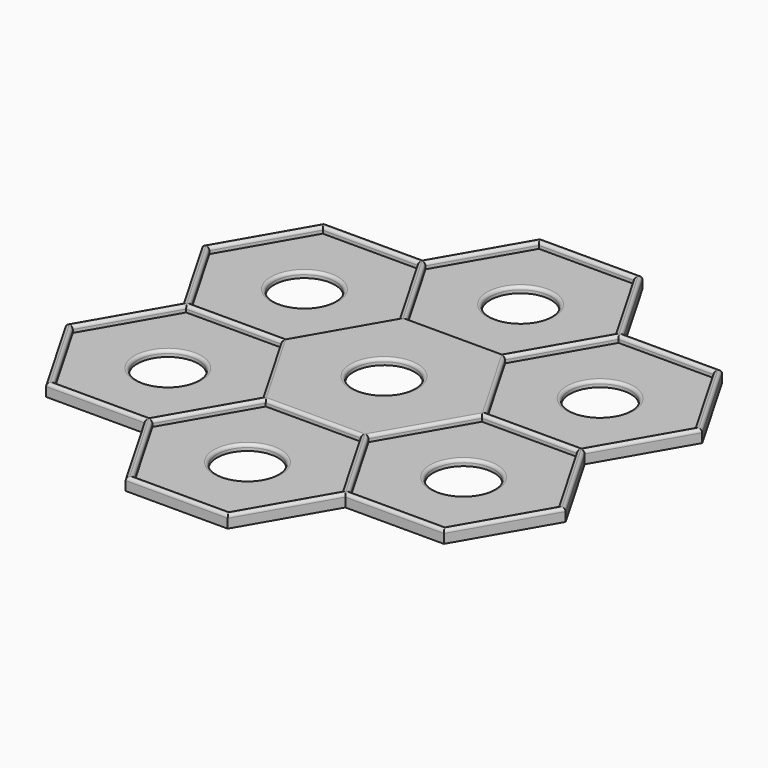
from build123d import *

# Parameters (mm, degrees)
F0_R     = 10
F1_DEPTH = 2
F2_DEPTH = 4
F3_R     = 0.99999
F4_START = 2
F4_DEPTH = 2
F5_R     = 1


# Not quite as in the source:
# - two fillets or chamfers of one size are made in one step
# - a fillet or chamfer is up to 0.001 mm smaller than in the source, because OpenCascade refuses the exact size


with BuildPart() as f1:
    # F0 (on Top) → F1 (new body)
    with BuildSketch(Plane.XY):
        Polygon((-64.0859146607, 54.9999594737), (-79.6743548546, 27.999949616), (-64.0858805124, 0.9999594737), (-32.9089659762, 0.9999791892), (-17.3205257822, 27.9999890469), (-32.9090001244, 54.9999791892), align=None)
        with Locations((-48.4974403184, 27.9999693314)):
            Circle(F0_R, mode=Mode.SUBTRACT)
    extrude(amount=F1_DEPTH)



with BuildPart() as f1b:
    # F0 (on Top) → F1, piece 2 (new body)
    with BuildSketch(Plane.XY):
        Polygon((-15.5885097552, 82.9999901422), (-31.1769499492, 55.9999802845), (-15.588475607, 28.9999901422), (15.5884389292, 29.0000098577), (31.1768791232, 56.0000197155), (15.588404781, 83.0000098577), align=None)
        with Locations((-3.5413e-05, 56)):
            Circle(F0_R, mode=Mode.SUBTRACT)
    extrude(amount=F1_DEPTH)


with BuildPart() as f1c:
    # F0 (on Top) → F1, piece 3 (new body)
    with BuildSketch(Plane.XY):
        Polygon((32.9089305632, 55.0000208108), (17.3204903692, 28.000010953), (32.9089647114, 1.0000208108), (64.0858792477, 1.0000405263), (79.6743194417, 28.000050384), (64.0858450994, 55.0000405263), align=None)
        with Locations((48.4974049054, 28.0000306685)):
            Circle(F0_R, mode=Mode.SUBTRACT)
    extrude(amount=F1_DEPTH)


with BuildPart() as f1d:
    # F0 (on Top) → F1, piece 4 (new body)
    with BuildSketch(Plane.XY):
        Polygon((32.9089659762, -0.9999791892), (17.3205257822, -27.9999890469), (32.9090001244, -54.9999791892), (64.0859146607, -54.9999594737), (79.6743548546, -27.999949616), (64.0858805124, -0.9999594737), align=None)
        with Locations((48.4974403184, -27.9999693314)):
            Circle(F0_R, mode=Mode.SUBTRACT)
    extrude(amount=F1_DEPTH)


with BuildPart() as f1e:
    # F0 (on Top) → F1, piece 5 (new body)
    with BuildSketch(Plane.XY):
        Polygon((-15.5884389292, -29.0000098577), (-31.1768791232, -56.0000197155), (-15.588404781, -83.0000098577), (15.5885097552, -82.9999901422), (31.1769499492, -55.9999802845), (15.588475607, -28.9999901422), align=None)
        with Locations((3.5413e-05, -56)):
            Circle(F0_R, mode=Mode.SUBTRACT)
    extrude(amount=F1_DEPTH)


with BuildPart() as f1f:
    # F0 (on Top) → F1, piece 6 (new body)
    with BuildSketch(Plane.XY):
        Polygon((-64.0858792477, -1.0000405263), (-79.6743194417, -28.000050384), (-64.0858450994, -55.0000405263), (-32.9089305632, -55.0000208108), (-17.3204903692, -28.000010953), (-32.9089647114, -1.0000208108), align=None)
        with Locations((-48.4974049054, -28.0000306685)):
            Circle(F0_R, mode=Mode.SUBTRACT)
    extrude(amount=F1_DEPTH)


with BuildPart() as f1_1:
    add(f1.part)

    add(f1b.part)  # F2 merges F1b

    add(f1c.part)  # F2 merges F1c

    add(f1d.part)  # F2 merges F1d

    add(f1e.part)  # F2 merges F1e

    add(f1f.part)  # F2 merges F1f
    # F0 (on Top) → F2 (join)
    with BuildSketch(Plane.XY):
        Polygon((-81.9837559314, 27.9999481555), (-65.8179547179, 0), (-81.9837445487, -28.0000102228), (-65.2405443731, -57.0000412565), (-32.9089292984, -57.0000208108), (-16.7431040546, -85.0000105879), (16.7432115584, -84.999989412), (32.9090013892, -56.9999791892), (65.2406164638, -56.9999587435), (81.9837559314, -27.9999481555), (65.8179306876, 4.16216e-05), (81.9837205184, 28.0000518444), (65.2405443731, 57.0000412565), (32.9089292984, 57.0000208108), (16.7431040546, 85.0000105879), (-16.7432115584, 84.999989412), (-32.9090013892, 56.9999791892), (-65.2406164638, 56.9999587435), align=None)
        Polygon((-64.0858450994, -55.0000405263), (-79.6743194417, -28.000050384), (-64.0858792477, -1.0000405263), (-32.9089647114, -1.0000208108), (-17.3204903692, -28.000010953), (-32.9089305632, -55.0000208108), align=None, mode=Mode.SUBTRACT)
        Polygon((-15.5884743422, 26.9999901422), (15.588440194, 27.0000098577), (31.1769145362, 1.97155e-05), (15.5884743422, -26.9999901422), (-15.588440194, -27.0000098577), (-31.1769145362, -1.97155e-05), align=None, mode=Mode.SUBTRACT)
        Polygon((-15.588404781, -83.0000098577), (-31.1768791232, -56.0000197155), (-15.5884389292, -29.0000098577), (15.588475607, -28.9999901422), (31.1769499492, -55.9999802845), (15.5885097552, -82.9999901422), align=None, mode=Mode.SUBTRACT)
        Polygon((32.9090001244, -54.9999791892), (17.3205257822, -27.9999890469), (32.9089659762, -0.9999791892), (64.0858805124, -0.9999594737), (79.6743548546, -27.999949616), (64.0859146607, -54.9999594737), align=None, mode=Mode.SUBTRACT)
        Polygon((-64.0858805124, 0.9999594737), (-79.6743548546, 27.999949616), (-64.0859146607, 54.9999594737), (-32.9090001244, 54.9999791892), (-17.3205257822, 27.9999890469), (-32.9089659762, 0.9999791892), align=None, mode=Mode.SUBTRACT)
        Polygon((-15.588475607, 28.9999901422), (-31.1769499492, 55.9999802845), (-15.5885097552, 82.9999901422), (15.588404781, 83.0000098577), (31.1768791232, 56.0000197155), (15.5884389292, 29.0000098577), align=None, mode=Mode.SUBTRACT)
        Polygon((32.9089647114, 1.0000208108), (17.3204903692, 28.000010953), (32.9089305632, 55.0000208108), (64.0858450994, 55.0000405263), (79.6743194417, 28.000050384), (64.0858792477, 1.0000405263), align=None, mode=Mode.SUBTRACT)
    extrude(amount=F2_DEPTH)

    # F3 (radius 1 in the source; OpenCascade refuses exactly that, so slightly less here)
    f3_edges = [f1_1.edges().sort_by_distance(p)[0] for p in [
        (-9.999965, -56, 2),
        (-58.497405, -28.000031, 2),
        (-58.49744, 27.999969, 2),
        (-10.000035, 56, 2),
        (38.497405, 28.000031, 2),
        (38.49744, -27.999969, 2),
        (-48.497422, -1.000031, 4),
        (-71.880099, -14.500045, 4),
        (-71.880082, -41.500045, 4),
        (-48.497388, -55.000031, 4),
        (-25.11471, -41.500016, 4),
        (-25.114728, -14.500016, 4),
        (24.826017, 71.000016, 4),
        (-5.4e-05, 85, 4),
        (-24.826106, 70.999984, 4),
        (-49.074809, 56.999969, 4),
        (-73.612186, 42.499953, 4),
        (-73.900855, 13.999974, 4),
        (-73.90085, -14.000005, 4),
        (-73.612144, -42.500026, 4),
        (-49.074737, -57.000031, 4),
        (-24.826017, -71.000016, 4),
        (5.4e-05, -85, 4),
        (24.826106, -70.999984, 4),
        (49.074809, -56.999969, 4),
        (73.612186, -42.499953, 4),
        (73.900843, -13.999953, 4),
        (73.900826, 14.000047, 4),
        (73.612132, 42.500047, 4),
        (49.074737, 57.000031, 4),
        (-23.382642, -69.500015, 4),
        (-23.382659, -42.500015, 4),
        (1.8e-05, -29, 4),
        (23.382713, -42.499985, 4),
        (23.38273, -69.499985, 4),
        (5.2e-05, -83, 4),
        (71.880135, -41.499955, 4),
        (48.497457, -54.999969, 4),
        (25.114763, -41.499984, 4),
        (25.114746, -14.499984, 4),
        (48.497423, -0.999969, 4),
        (71.880118, -14.499955, 4),
        (-48.497423, 0.999969, 4),
        (-71.880118, 14.499955, 4),
        (-71.880135, 41.499955, 4),
        (-48.497457, 54.999969, 4),
        (-25.114763, 41.499984, 4),
        (-25.114746, 14.499984, 4),
        (-1.8e-05, 29, 4),
        (-23.382713, 42.499985, 4),
        (-23.38273, 69.499985, 4),
        (-5.2e-05, 83, 4),
        (23.382642, 69.500015, 4),
        (23.382659, 42.500015, 4),
        (25.114728, 14.500016, 4),
        (25.11471, 41.500016, 4),
        (48.497388, 55.000031, 4),
        (71.880082, 41.500045, 4),
        (71.880099, 14.500045, 4),
        (48.497422, 1.000031, 4),
    ]]
    fillet(f3_edges, radius=F3_R)

    # F0 (on Top) → F4 (join)
    with BuildSketch(Plane.XY.offset(F4_START)):
        Polygon((31.1769145362, 1.97155e-05), (15.588440194, 27.0000098577), (-15.5884743422, 26.9999901422), (-31.1769145362, -1.97155e-05), (-15.588440194, -27.0000098577), (15.5884743422, -26.9999901422), align=None)
        Circle(F0_R, mode=Mode.SUBTRACT)
    extrude(amount=F4_DEPTH)

    # F5
    f5_edges = [f1_1.edges().sort_by_distance(p)[0] for p in [
        (-10, 0, 4),
    ]]
    fillet(f5_edges, radius=F5_R)


solid = f1_1.part
